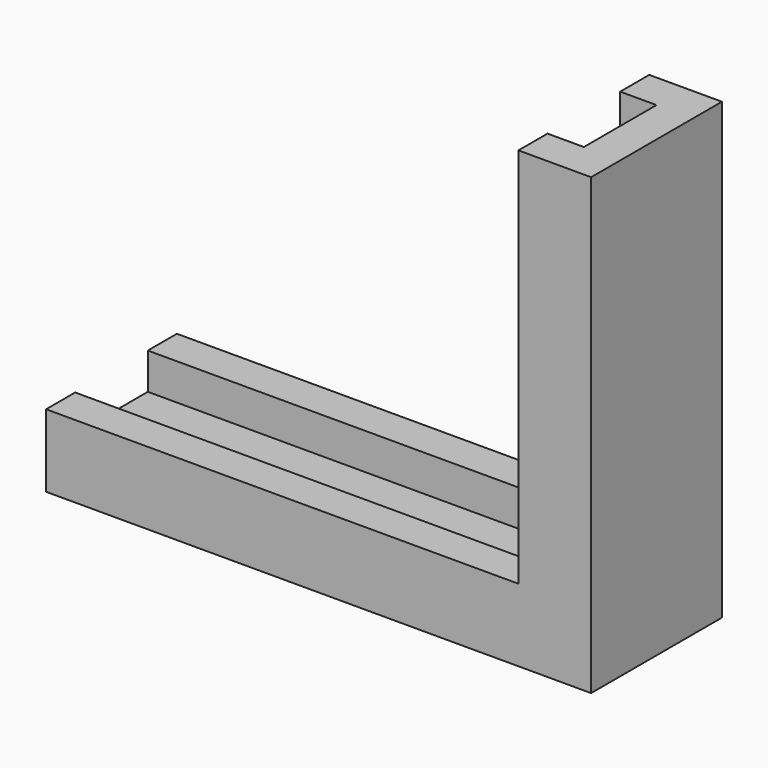
from build123d import *

# Parameters (mm, degrees)
F0_W     = 2
F0_H     = 5
F0_W_2   = 26
F0_H_2   = 2
F1_DEPTH = 2
F2_DEPTH = 4
F3_DEPTH = 25


with BuildPart() as f1:
    # F0 (on Top) → F1 (new body)
    with BuildSketch(Plane.XY):
        Polygon((11, -4.5), (15, -4.5), (15, -2.5), (13, -2.5), (11, -2.5), align=None)
        Polygon((-15, -4.5), (11, -4.5), (11, -2.5), (-13.6096680164, -2.5), (-15, -2.5), align=None)
        with Locations((14, 0)):
            Rectangle(F0_W, F0_H)
        with Locations((12, 0)):
            Rectangle(F0_W, F0_H)
        Polygon((-13.6096680164, -2.5), (11, -2.5), (11, 2.5), (-15, 2.5), (-15, -2.5), align=None)
        Polygon((13, 2.5), (15, 2.5), (15, 4.5), (11, 4.5), (11, 2.5), align=None)
        with Locations((-2, 3.5)):
            Rectangle(F0_W_2, F0_H_2)
    extrude(amount=F1_DEPTH)

    # F0 (on Top) → F2 (join)
    with BuildSketch(Plane.XY):
        Polygon((11, -4.5), (15, -4.5), (15, -2.5), (13, -2.5), (11, -2.5), align=None)
        Polygon((-15, -4.5), (11, -4.5), (11, -2.5), (-13.6096680164, -2.5), (-15, -2.5), align=None)
        with Locations((14, 0)):
            Rectangle(F0_W, F0_H)
        Polygon((13, 2.5), (15, 2.5), (15, 4.5), (11, 4.5), (11, 2.5), align=None)
        with Locations((-2, 3.5)):
            Rectangle(F0_W_2, F0_H_2)
    extrude(amount=F2_DEPTH)

    # F0 (on Top) → F3 (join)
    with BuildSketch(Plane.XY):
        with Locations((14, 0)):
            Rectangle(F0_W, F0_H)
        Polygon((11, -4.5), (15, -4.5), (15, -2.5), (13, -2.5), (11, -2.5), align=None)
        Polygon((13, 2.5), (15, 2.5), (15, 4.5), (11, 4.5), (11, 2.5), align=None)
    extrude(amount=F3_DEPTH)


solid = f1.part
